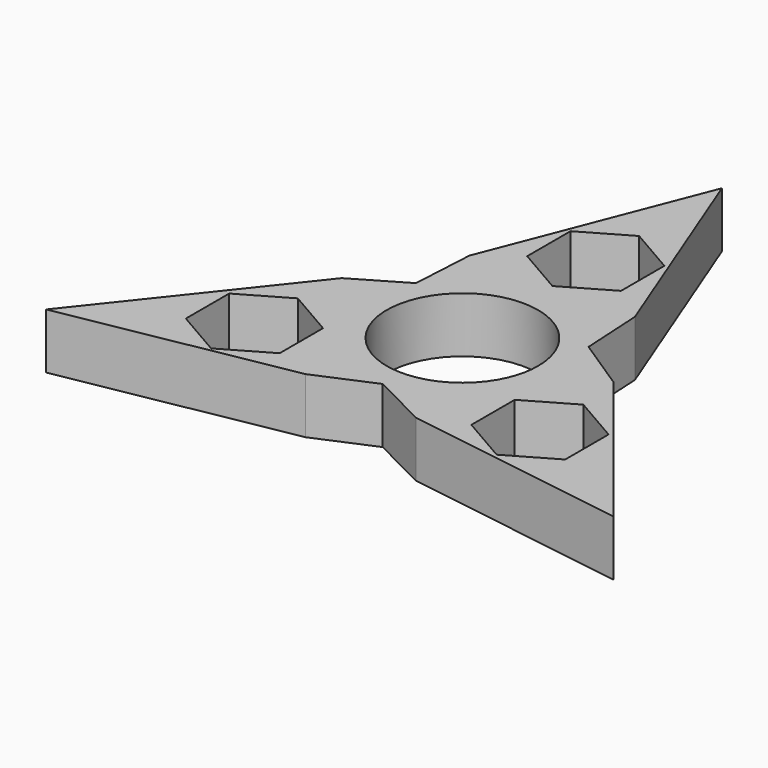
from build123d import *

# Parameters (mm, degrees)
F1_DEPTH = 8


# Not quite as in the source:
# - ends of sketch curves that miss each other by under 0.0002 mm in the source are joined


with BuildPart() as f1:
    # F0 (on Top) → F1 (new body)
    with BuildSketch(Plane.XY):
        Polygon((8.0340162625, -18.397915233), (40.4422496394, -23.3490666912), (19.9500470696, 2.2415004228), (12.4201863904, 7.1707647293), (11.9161368405, 16.1565585761), (0, 46.6985489201), (-11.9161368405, 16.1565585761), (-12.4201318249, 7.170681376), (-19.702678316, 2.9058864326), (-40.8897429157, -23.8067811423), (-8.2744899158, -17.8816622036), (0, -14.3414903669), align=None)
        Polygon((-20.4809666485, -4.0247617542), (-13.725968499, -7.9247617542), (-13.725968499, -15.7247617542), (-20.4809666485, -19.6247617542), (-27.2359647981, -15.7247617542), (-27.2359647981, -7.9247617542), align=None, mode=Mode.SUBTRACT)
        Polygon((13.9923272284, -15.8783317751), (13.9923272284, -8.0783317751), (20.7473253779, -4.1783317751), (27.5023235274, -8.0783317751), (27.5023235274, -15.8783317751), (20.7473253779, -19.7783317751), align=None, mode=Mode.SUBTRACT)
        with BuildLine():
            ThreePointArc((-9.4396629017, -5.4500242478), (-2.8211411141, 10.5285878832), (10.9, 0))
            ThreePointArc((10.9, 0), (10.5285987532, -2.8211005467), (9.4397049001, -5.4499515043))
            ThreePointArc((9.4397049001, -5.4499515043), (4.19985e-05, -10.8999999999), (-9.4396629017, -5.4500242478))
        make_face(mode=Mode.SUBTRACT)
        Polygon((6.7549981495, 27.9), (6.7549981495, 20.1), (0, 16.2), (-6.7549981495, 20.1), (-6.7549981495, 27.9), (0, 31.8), align=None, mode=Mode.SUBTRACT)
    extrude(amount=F1_DEPTH)


solid = f1.part
